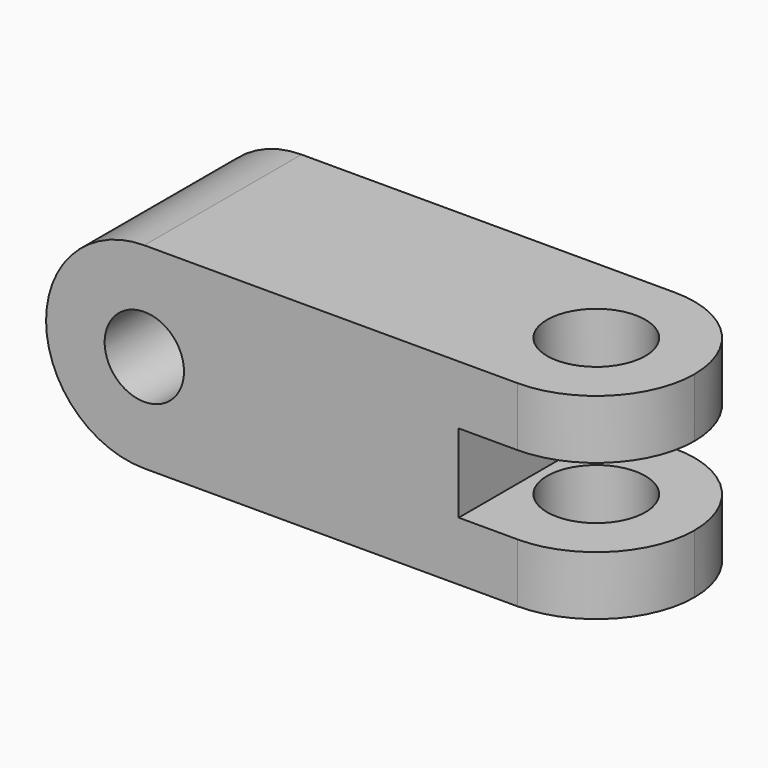
from build123d import *

# Parameters (mm, degrees)
F0_R     = 6.4084954246
F1_DEPTH = 31.75
F3_D     = 15.875
F4_R     = 15.87499


# Not quite as in the source:
# - a fillet or chamfer is up to 0.001 mm smaller than in the source, because OpenCascade refuses the exact size


with BuildPart() as f1:
    # F0 (on Front) → F1 (new body)
    with BuildSketch(Plane.XZ):
        with BuildLine():
            Line((32.4883715089, 9.525), (-43.7116284911, 9.525))
            ThreePointArc((-43.7116284911, 9.525), (-59.5866284911, -6.35), (-43.7116284911, -22.225))
            Line((-43.7116284911, -22.225), (32.4883715089, -22.225))
            Line((32.4883715089, -22.225), (32.4883715089, -12.7))
            Line((32.4883715089, -12.7), (7.0883715089, -12.7))
            Line((7.0883715089, -12.7), (7.0883715089, 0))
            Line((7.0883715089, 0), (32.4883715089, 0))
            Line((32.4883715089, 0), (32.4883715089, 9.525))
        make_face()
        with Locations((-43.7116284911, -6.35)):
            Circle(F0_R, mode=Mode.SUBTRACT)
    extrude(amount=F1_DEPTH)

    # F3 (through all)
    with Locations(Plane.XY.offset(9.525)):
        with Locations((16.6133715089, -15.875)):
            Hole(F3_D / 2)

    # F4 (radius 15.875 in the source; OpenCascade refuses exactly that, so slightly less here)
    f4_edges = [f1.edges().sort_by_distance(p)[0] for p in [
        (32.488372, -31.75, 4.7625),
        (32.488372, 0, 4.7625),
        (32.488372, -31.75, -17.4625),
        (32.488372, 0, -17.4625),
    ]]
    fillet(f4_edges, radius=F4_R)


solid = f1.part
